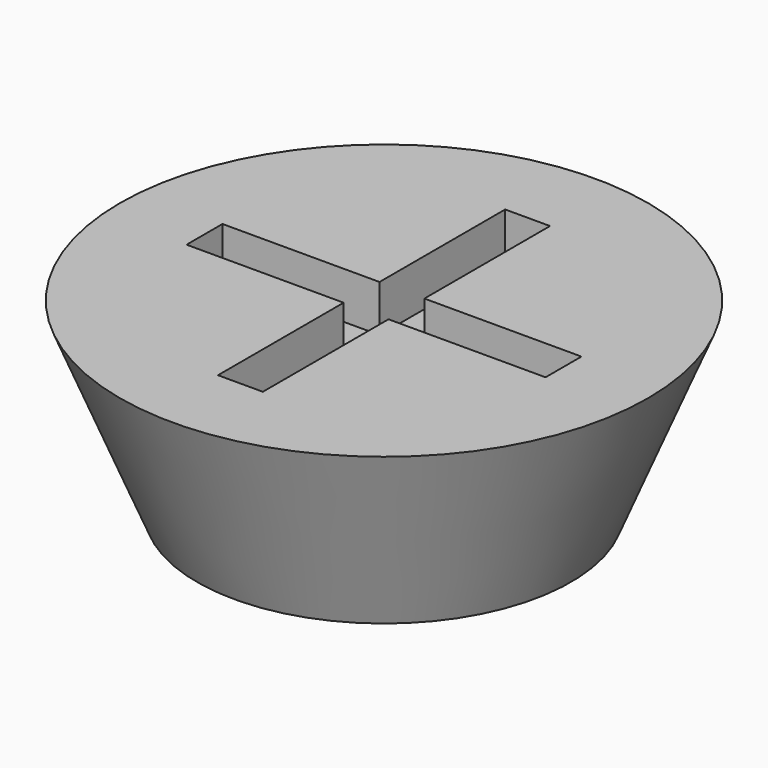
from build123d import *

# Parameters (mm, degrees)
F2_W     = 0.254
F2_H     = 0.889
F2_H_2   = 0.254
F2_W_2   = 0.889
F3_DEPTH = 0.2645833333


with BuildPart() as f1:
    # F0 (on Front) → F1 (revolve)
    with BuildSketch(Plane.XZ):
        Polygon((-1.0583333333, 0), (0, 0), (0, 1.0583333333), (-1.4950298937, 1.0583333333), align=None)
    revolve(axis=Axis((0, 0, 0.5291666667), (0, 0, -1)))

    # F2 (on face) → F3 (cut)
    with BuildSketch(Plane.XY.offset(1.0583333333)):
        with Locations((0, 0.5715)):
            Rectangle(F2_W, F2_H)
        Rectangle(F2_W, F2_H_2)
        with Locations((-0.5715, 0)):
            Rectangle(F2_W_2, F2_H_2)
        with Locations((0, -0.5715)):
            Rectangle(F2_W, F2_H)
        with Locations((0.5715, 0)):
            Rectangle(F2_W_2, F2_H_2)
    extrude(amount=-F3_DEPTH, mode=Mode.SUBTRACT)


solid = f1.part
